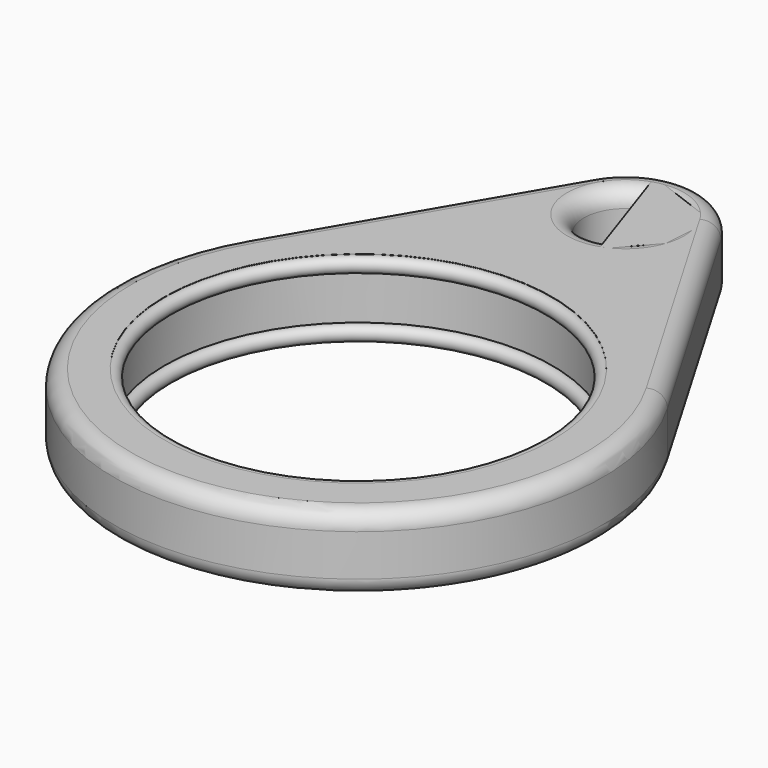
from build123d import *

# Parameters (mm, degrees)
F0_R     = 11.6
F0_R_2   = 2.5
F1_DEPTH = 4.5
F2_R     = 0.99999
F3_R     = 0.45


# Not quite as in the source:
# - a fillet or chamfer is up to 0.001 mm smaller than in the source, because OpenCascade refuses the exact size


with BuildPart() as f1:
    # F0 (on Top) → F1 (new body)
    with BuildSketch(Plane.XY):
        with BuildLine():
            ThreePointArc((3.8840370428, 22.2725), (0, 24.5), (-3.8840370428, 22.2725))
            Line((-3.8840370428, 22.2725), (-12.6015424056, 7.373))
            ThreePointArc((-12.6015424056, 7.373), (0, -14.6), (12.6015424056, 7.373))
            Line((12.6015424056, 7.373), (3.8840370428, 22.2725))
        make_face()
        Circle(F0_R, mode=Mode.SUBTRACT)
        with Locations((0, 20)):
            Circle(F0_R_2, mode=Mode.SUBTRACT)
    extrude(amount=F1_DEPTH)

    # F2 (radius 1 in the source; OpenCascade refuses exactly that, so slightly less here)
    f2_edges = [f1.edges().sort_by_distance(p)[0] for p in [
        (-2.5, 20, 4.5),
        (-2.5, 20, 0),
        (0, -14.6, 4.5),
        (8.24279, 14.82275, 0),
    ]]
    fillet(f2_edges, radius=F2_R)

    # F3 (on Front) → F4 (revolve)
    with BuildSketch(Plane.XZ):
        with Locations((11.5, 4.05)):
            Circle(F3_R)
        with Locations((11.5, 0.45)):
            Circle(F3_R)
    revolve(axis=Axis((0, 0, 3.4984555226), (0, 0, -1)))


solid = f1.part
